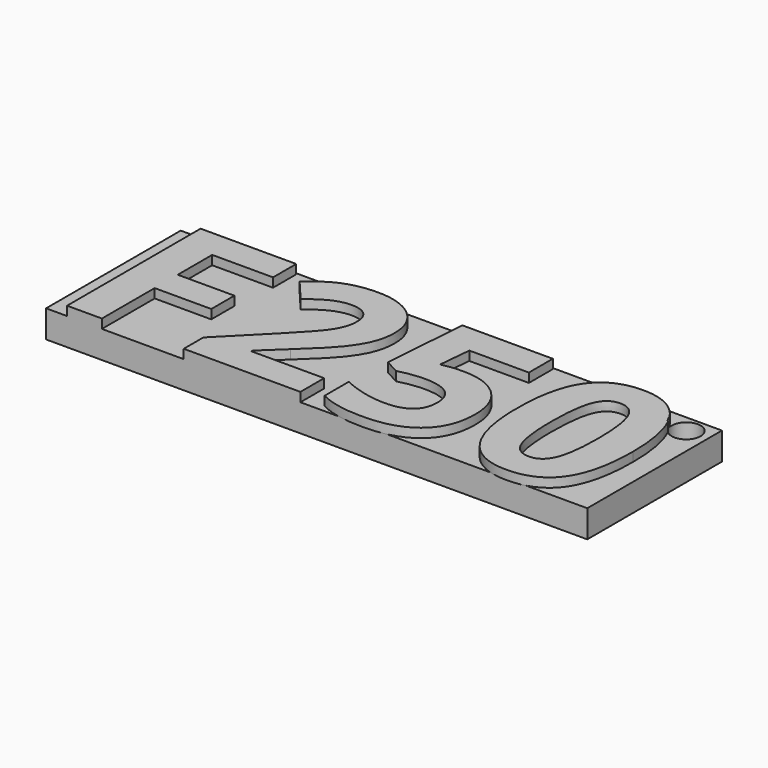
from build123d import *

# Parameters (mm, degrees)
F0_W         = 75.1956477761
F0_H         = 23.3840115834
F1_DEPTH     = 3.81
F2_TEXT_SIZE = 32.4777938658
F3_DEPTH     = 1.27
F4_R         = 2.0086139444
F5_DEPTH     = 20.1168


# Not quite as in the source:
# - Text() gives the source's letters only with a copy of the font that has no kerning and outlines rounded to 1/6400 em; it was checked with that copy


with BuildPart() as f1:
    # F0 (on Top) → F1 (new body)
    with BuildSketch(Plane.XY):
        with Locations((2.1779239178, 13.8699285453)):
            Rectangle(F0_W, F0_H)
    extrude(amount=F1_DEPTH)

    # F2 (on face) → F3 (join)
    with BuildSketch(Plane.XY.offset(3.81)):
        with Locations((-35.4198999703, 2.1779227536)):
            Text('F250', F2_TEXT_SIZE, font='Open Sans', font_style=FontStyle.BOLD, text_align=(TextAlign.LEFT, TextAlign.BOTTOM))
    extrude(amount=F3_DEPTH)

    # F4 (on face) → F5 (cut)
    with BuildSketch(Plane.XY.offset(5.08)):
        with Locations((36.8030145764, 23.0731870979)):
            Circle(F4_R)
    extrude(amount=-F5_DEPTH, mode=Mode.SUBTRACT)


solid = f1.part
